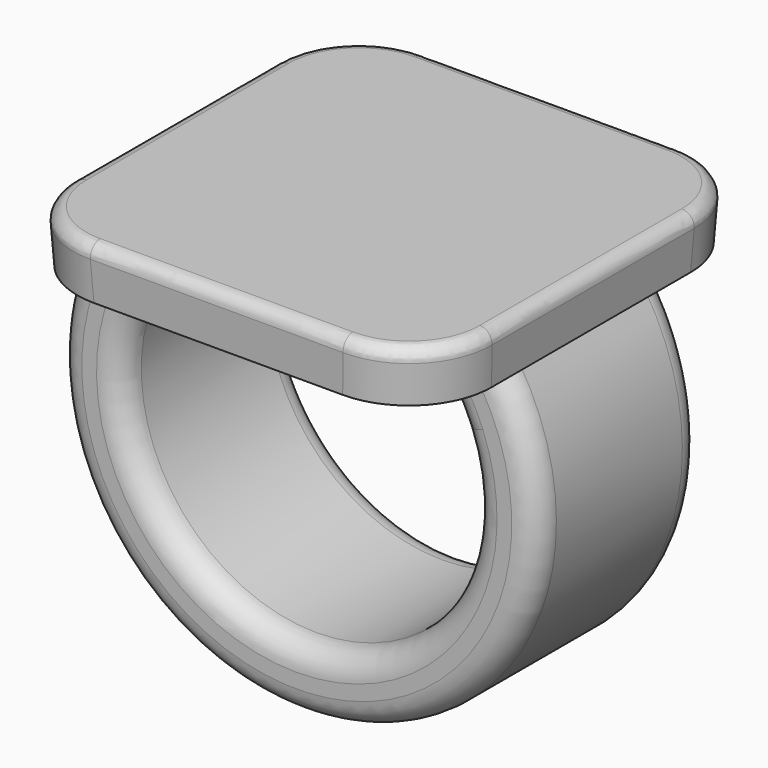
from build123d import *

# Parameters (mm, degrees)
F0_W          = 25.4
F0_H          = 25.4
F1_DEPTH      = 3.175
F1_TAPER      = -3
F3_W          = 5.08
F3_H          = 12.7
F6_DEPTH      = 6.35
F6_DEPTH_BACK = 6.35
F7_R          = 5.08
F8_R          = 1.524
F9_R          = 0.762


with BuildPart() as f1:
    # F0 (on Top) → F1 (new body)
    with BuildSketch(Plane.XY):
        Rectangle(F0_W, F0_H)
    extrude(amount=F1_DEPTH, taper=F1_TAPER)

    # F4: sweep along a path in F2
    with BuildLine(Plane.XZ) as f4_path:
        ThreePointArc((-11.781251058, 0), (-0.2676574513, -21.7919597056), (11.2459361553, 0))
    # F3 (on face) → F4 (sweep)
    with BuildSketch(Plane(origin=(0, 0, 0), x_dir=(1, 0, 0), z_dir=(0, 0, -1))):
        with Locations((-10.16, 0)):
            Rectangle(F3_W, F3_H)
    sweep(path=f4_path.line)

    # F5 (on Front) → F6 (join, two sides)
    with BuildSketch(Plane.XZ) as f6_sk:
        with BuildLine():
            ThreePointArc((7.0846850973, 0), (8.6199219464, -1.7914332396), (9.727769055, -3.8744262831))
            Line((9.727769055, -3.8744262831), (11.2459361553, 0))
            Line((11.2459361553, 0), (7.0846850973, 0))
        make_face()
    extrude(amount=F6_DEPTH)
    extrude(f6_sk.sketch, amount=-F6_DEPTH_BACK)

    # F7
    f7_edges = [f1.edges().sort_by_distance(p)[0] for p in [
        (12.783197, -12.783197, 1.5875),
        (-12.783197, -12.783197, 1.5875),
        (-12.783197, 12.783197, 1.5875),
        (12.783197, 12.783197, 1.5875),
    ]]
    fillet(f7_edges, radius=F7_R)

    # F8
    f8_edges = [f1.edges().sort_by_distance(p)[0] for p in [
        (-2.612709, -6.35, -18.354411),
        (8.619922, -6.35, -1.791433),
        (-2.612709, 6.35, -18.354411),
        (-0.267657, -6.35, -22.560042),
        (-0.267657, 6.35, -22.560042),
        (8.619922, 6.35, -1.791433),
    ]]
    fillet(f8_edges, radius=F8_R)

    # F9
    f9_edges = [f1.edges().sort_by_distance(p)[0] for p in [
        (0, -12.866395, 3.175),
        (-11.381378, -11.381378, 3.175),
        (11.381378, -11.381378, 3.175),
        (-12.866395, 0, 3.175),
        (12.866395, 0, 3.175),
        (-11.381378, 11.381378, 3.175),
        (11.381378, 11.381378, 3.175),
        (0, 12.866395, 3.175),
    ]]
    fillet(f9_edges, radius=F9_R)


solid = f1.part
